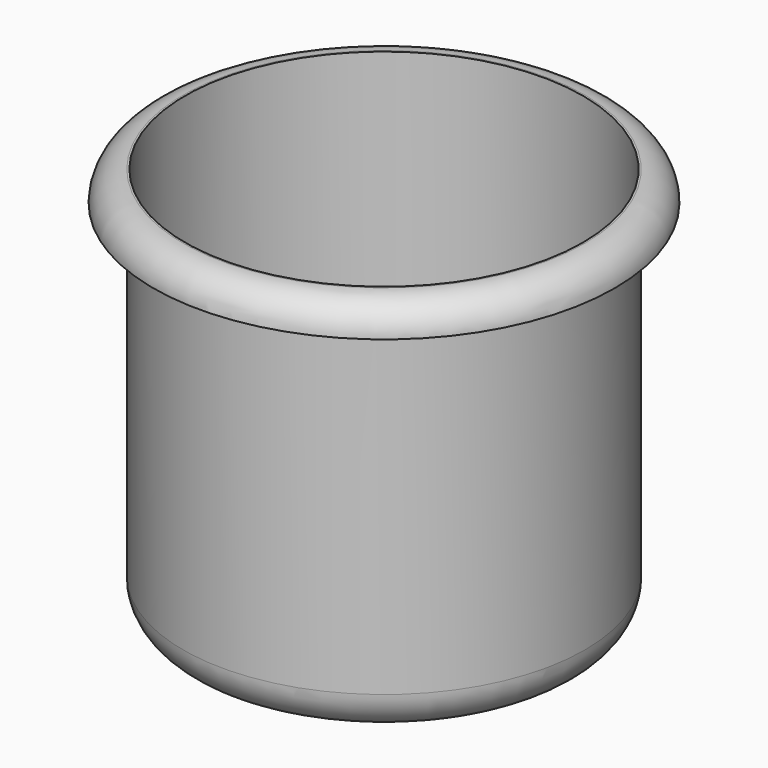
from build123d import *

# Parameters (mm, degrees)
F0_R     = 101
F1_DEPTH = 200
F2_R     = 20
F3_R     = 100
F4_DEPTH = 180
F5_R     = 116
F5_R_2   = 101
F6_DEPTH = 15
F7_R     = 14.99999


# Not quite as in the source:
# - a fillet or chamfer is up to 0.001 mm smaller than in the source, because OpenCascade refuses the exact size


with BuildPart() as f1:
    # F0 (on Top) → F1 (new body)
    with BuildSketch(Plane.XY):
        Circle(F0_R)
    extrude(amount=F1_DEPTH)

    # F2
    f2_edges = [f1.edges().sort_by_distance(p)[0] for p in [
        (-101, 0, 0),
    ]]
    fillet(f2_edges, radius=F2_R)

    # F3 (on face) → F4 (cut)
    with BuildSketch(Plane.XY.offset(200)):
        Circle(F3_R)
    extrude(amount=-F4_DEPTH, mode=Mode.SUBTRACT)

    # F5 (on face) → F6 (join)
    with BuildSketch(Plane.XY.offset(200)):
        Circle(F5_R)
        Circle(F5_R_2, mode=Mode.SUBTRACT)
    extrude(amount=-F6_DEPTH)

    # F7 (radius 15 in the source; OpenCascade refuses exactly that, so slightly less here)
    f7_edges = [f1.edges().sort_by_distance(p)[0] for p in [
        (-116, 0, 200),
    ]]
    fillet(f7_edges, radius=F7_R)


solid = f1.part
